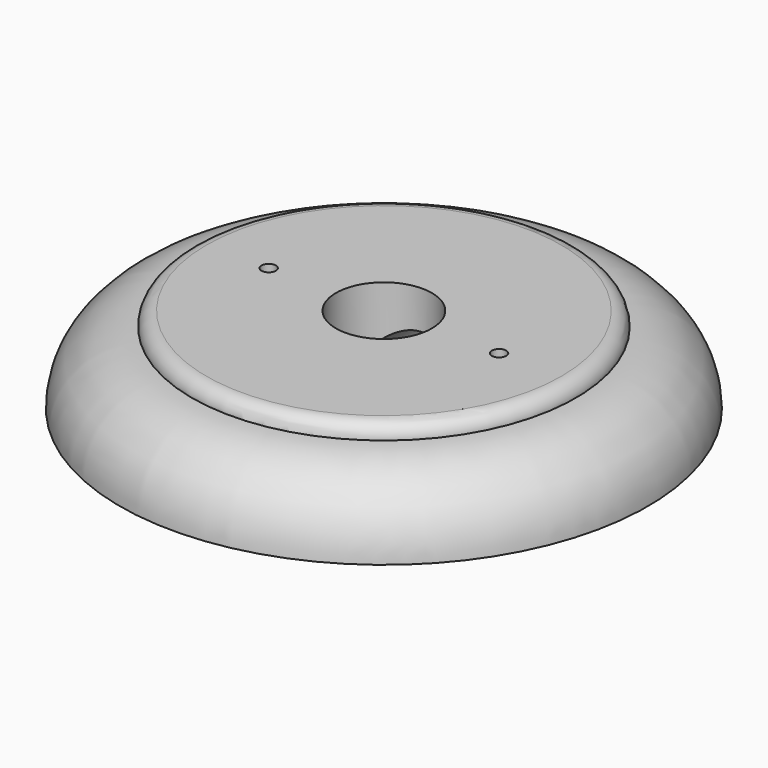
from build123d import *

# Parameters (mm, degrees)
F0_W     = 10
F0_H     = 25.0418604054
F0_H_2   = 18
F0_H_3   = 6.9581395946
F3_R     = 10
F4_DEPTH = 141.6
F7_D     = 3
F8_D     = 3
F9_R     = 2.99999


# Not quite as in the source:
# - a fillet or chamfer that OpenCascade refuses, or shapes differently, is made with other operations: its cross-section is extruded or revolved along the edge and cut away or added
# - a fillet or chamfer is up to 0.001 mm smaller than in the source, because OpenCascade refuses the exact size


with BuildPart() as f1:
    # F0 (on Front) → F1 (revolve)
    with BuildSketch(Plane.XZ):
        Polygon((-55, 15), (-55, 0), (0, 0), (0, 18), (-40, 18), (-40, 15), align=None)
    revolve(axis=Axis((0, 0, 9), (0, 0, 1)))

    # F0 (on Front) → F2 (revolve, cut)
    with BuildSketch(Plane.XZ):
        with Locations((5, 30.5209302027)):
            Rectangle(F0_W, F0_H)
        with Locations((5, 9)):
            Rectangle(F0_W, F0_H_2)
        with Locations((5, -3.4790697973)):
            Rectangle(F0_W, F0_H_3)
    revolve(axis=Axis((0, 0, 18.0418604054), (0, 0, 1)), mode=Mode.SUBTRACT)

    # F3 (on Front) → F4 (cut)
    with BuildSketch(Plane.XZ):
        Circle(F3_R)
    extrude(amount=-F4_DEPTH, mode=Mode.SUBTRACT)

    # F5: fillet of radius 15 on 1 edges, made by hand

    # F5_s1 → F5_t2 (revolve, cut)
    with BuildSketch(Plane.XZ):
        with BuildLine():
            ThreePointArc((-55, 0), (-50.6066017178, 10.6066017178), (-40, 15))
            Line((-40, 15), (-55, 15))
            Line((-55, 15), (-55, 0))
        make_face()
    revolve(axis=Axis((0, 0, 15), (0, 0, 1)), mode=Mode.SUBTRACT)

    # F7 (through all)
    with Locations(Plane(origin=(0, 0, 0), x_dir=(1, 0, 0), z_dir=(0, 0, -1))):
        with Locations((24, 0)):
            Hole(F7_D / 2)

    # F8 (through all)
    with Locations(Plane(origin=(0, 0, 0), x_dir=(1, 0, 0), z_dir=(0, 0, -1))):
        with Locations((-24, 0)):
            Hole(F8_D / 2)

    # F9 (radius 3 in the source; OpenCascade refuses exactly that, so slightly less here)
    f9_edges = [f1.edges().sort_by_distance(p)[0] for p in [
        (40, 0, 18),
    ]]
    fillet(f9_edges, radius=F9_R)


solid = f1.part
